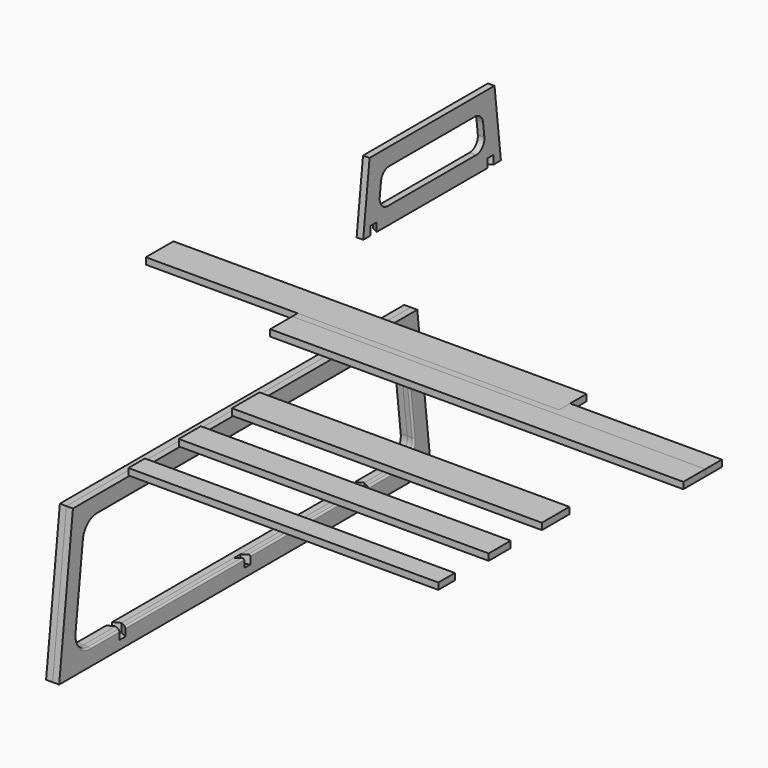
from build123d import *

# Parameters (mm, degrees)
F0_W          = 1200
F0_H          = 60
F1_DEPTH      = 19
F2_W          = 1200
F2_H          = 80
F3_DEPTH      = 19
F4_W          = 1200
F4_H          = 100
F5_DEPTH      = 19
F7_DEPTH      = 19
F8_DEPTH      = 19
F10_DEPTH     = 25
F12_DEPTH     = 25
F14_DEPTH     = 25
F16_DEPTH     = 25
F18_R         = 6.35
F19_DEPTH     = 10
F20_R         = 3.1
F21_DEPTH     = 571.5798048431
F22_R         = 6.35
F22_R_2       = 3.1
F23_DEPTH     = 10
F24_R         = 6.35
F25_DEPTH     = 10
F27_DEPTH     = 25
F28_DEPTH     = 25
F30_DEPTH     = 19
F32_DEPTH     = 25
F33_W         = 900
F33_H         = 60
F34_DEPTH     = 19
F33_H_2       = 80
F35_DEPTH     = 19
F33_H_3       = 100
F36_DEPTH     = 19
F37_T1_DEPTH  = 456.85740495
F37_T3_DEPTH  = 429.8821422275
F37_T5_DEPTH  = 128.89740651
F37_T7_DEPTH  = 118.9306462831
F37_T9_DEPTH  = 231.5496739088
F37_T11_DEPTH = 1071.9082714241
F37_T13_DEPTH = 231.5496739088
F37_T16_ANGLE = 96.6325146151
F37_T18_ANGLE = 83.3674853849
F37_T20_ANGLE = 83.3674853849
F37_T22_ANGLE = 96.6325146151


# Not quite as in the source:
# - a fillet or chamfer that OpenCascade refuses, or shapes differently, is made with other operations: its cross-section is extruded or revolved along the edge and cut away or added
# - a feature names something its author has since deleted; it is built from what else it names


with BuildPart() as f1:
    # F0 (on Top) → F1 (new body)
    with BuildSketch(Plane.XY):
        with Locations((600, 30)):
            Rectangle(F0_W, F0_H)
    extrude(amount=F1_DEPTH)

    # F24 (on face) → F25 (cut)
    with BuildSketch(Plane(origin=(0, 0, -182.5788048431), x_dir=(1, 0, 0), z_dir=(0, 0, -1))):
        with Locations((9.5, 194.6265311424)):
            Circle(F24_R)
    extrude(amount=-F25_DEPTH, mode=Mode.SUBTRACT)


with BuildPart() as f3:
    # F2 (on Top) → F3 (new body)
    with BuildSketch(Plane.XY):
        with Locations((600, -40)):
            Rectangle(F2_W, F2_H)
    extrude(amount=F3_DEPTH)


with BuildPart() as f5:
    # F4 (on Top) → F5 (new body)
    with BuildSketch(Plane.XY):
        with Locations((159.0859787539, 69.8453307072)):
            Rectangle(F4_W, F4_H)
    extrude(amount=F5_DEPTH)


with BuildPart() as f7:
    # F6 (on Right) → F7 (new body)
    with BuildSketch(Plane.YZ):
        Polygon((430.3734688576, -132.5788048431), (-819.6265311424, -132.5788048431), (-869.6265311424, -562.5788048431), (480.3734688576, -562.5788048431), align=None)
        with BuildLine():
            ThreePointArc((-780.2460358695, -226.8037619344), (-763.8315905601, -195.2374594909), (-730.5806668544, -182.5788048431))
            Line((-730.5806668544, -182.5788048431), (341.3276045696, -182.5788048431))
            ThreePointArc((341.3276045696, -182.5788048431), (374.5785282753, -195.2374594909), (390.9929735847, -226.8037619344))
            Line((390.9929735847, -226.8037619344), (417.7371596312, -456.8037619344))
            ThreePointArc((417.7371596312, -456.8037619344), (405.4131359684, -495.8297285488), (368.0717906162, -512.5788048431))
            Line((368.0717906162, -512.5788048431), (-757.3248529009, -512.5788048431))
            ThreePointArc((-757.3248529009, -512.5788048431), (-794.6661982532, -495.8297285488), (-806.990221916, -456.8037619344))
            Line((-806.990221916, -456.8037619344), (-780.2460358695, -226.8037619344))
        make_face(mode=Mode.SUBTRACT)
    extrude(amount=F7_DEPTH)

    # F9 (on face) → F10 (cut)
    with BuildSketch(Plane.XY.offset(-132.5788048431)):
        Polygon((19, -176.7615311424), (0, -189.5771929624), (0, -212.495333984), (19, -199.679672164), align=None)
    extrude(amount=-F10_DEPTH, mode=Mode.SUBTRACT)

    # F11 (on face) → F12 (cut)
    with BuildSketch(Plane.XY.offset(-512.5788048431)):
        Polygon((45.0043368484, -157.1230627047), (-59.9762402534, -227.9333560629), (-53.8986982225, -246.7521432232), (55.6290020144, -172.8747765833), align=None)
    extrude(amount=-F12_DEPTH, mode=Mode.SUBTRACT)

    # F18 (on face) → F19 (cut)
    with BuildSketch(Plane(origin=(0, 0, -562.5788048431), x_dir=(1, 0, 0), z_dir=(0, 0, -1))):
        with Locations((9.5, 194.6265311424)):
            Circle(F18_R)
    extrude(amount=-F19_DEPTH, mode=Mode.SUBTRACT)

    # F20 (on face) → F21 (cut, through all)
    with BuildSketch(Plane(origin=(0, 0, -552.5788048431), x_dir=(1, 0, 0), z_dir=(0, 0, -1))):
        with Locations((9.5, 194.6265311424)):
            Circle(F20_R)
    extrude(amount=-F21_DEPTH, mode=Mode.SUBTRACT)

    # F22 (on face) → F23 (cut)
    with BuildSketch(Plane(origin=(0, 0, -182.5788048431), x_dir=(1, 0, 0), z_dir=(0, 0, -1))):
        with Locations((9.5, 194.6265311424)):
            Circle(F22_R)
        with Locations((9.5, 194.6265311424)):
            Circle(F22_R_2, mode=Mode.SUBTRACT)
    extrude(amount=-F23_DEPTH, mode=Mode.SUBTRACT)


with BuildPart() as f8:
    # F6 (on Right) → F8 (new body)
    with BuildSketch(Plane.YZ):
        Polygon((430.3734688576, -132.5788048431), (-819.6265311424, -132.5788048431), (-869.6265311424, -562.5788048431), (480.3734688576, -562.5788048431), align=None)
        with BuildLine():
            ThreePointArc((-780.2460358695, -226.8037619344), (-763.8315905601, -195.2374594909), (-730.5806668544, -182.5788048431))
            Line((-730.5806668544, -182.5788048431), (341.3276045696, -182.5788048431))
            ThreePointArc((341.3276045696, -182.5788048431), (374.5785282753, -195.2374594909), (390.9929735847, -226.8037619344))
            Line((390.9929735847, -226.8037619344), (417.7371596312, -456.8037619344))
            ThreePointArc((417.7371596312, -456.8037619344), (405.4131359684, -495.8297285488), (368.0717906162, -512.5788048431))
            Line((368.0717906162, -512.5788048431), (-757.3248529009, -512.5788048431))
            ThreePointArc((-757.3248529009, -512.5788048431), (-794.6661982532, -495.8297285488), (-806.990221916, -456.8037619344))
            Line((-806.990221916, -456.8037619344), (-780.2460358695, -226.8037619344))
        make_face(mode=Mode.SUBTRACT)
    extrude(amount=-F8_DEPTH)

    # F13 (on face) → F14 (cut)
    with BuildSketch(Plane(origin=(0, 0, -562.5788048431), x_dir=(1, 0, 0), z_dir=(0, 0, -1))):
        Polygon((0, 212.4915311424), (-19, 199.6758693224), (-19, 176.7577283008), (0, 189.5733901208), align=None)
    extrude(amount=-F14_DEPTH, mode=Mode.SUBTRACT)

    # F15 (on face) → F16 (cut)
    with BuildSketch(Plane(origin=(0, 0, -182.5788048431), x_dir=(1, 0, 0), z_dir=(0, 0, -1))):
        Polygon((0, 212.4915311424), (-19, 199.6758693224), (-19, 176.7577283008), (0, 189.5733901208), align=None)
    extrude(amount=-F16_DEPTH, mode=Mode.SUBTRACT)


with BuildPart() as f27_tool:
    # F26 (on face) → F27 (new body)
    with BuildSketch(Plane.XY.offset(-512.5788048431)):
        Polygon((0, -619.4719911424), (0, -640.9274424049), (19, -650.8942066179), (19, -629.4387553554), align=None)
        Polygon((-87.6130647374, -686.8863244162), (0, -640.9274424049), (0, -619.4719911424), (-87.6130647374, -665.4308731537), align=None)
        Polygon((0, 261.6411483192), (0, 240.1856970567), (19, 230.2189328437), (19, 251.6743841062), align=None)
    extrude(amount=-F27_DEPTH)


with BuildPart() as f7_1:
    add(f7.part)

    # F27: cut by f27_tool
    add(f27_tool.part, mode=Mode.SUBTRACT)

    # F37: fillet of radius 5 on 11 edges, made by hand

    # F37_s2 → F37_t1 (cut)
    with BuildSketch(Plane.XZ.offset(185.0813504054)):
        with BuildLine():
            ThreePointArc((19, -517.5788048431), (17.5355339059, -514.0432709372), (14, -512.5788048431))
            Line((14, -512.5788048431), (19, -512.5788048431))
            Line((19, -512.5788048431), (19, -517.5788048431))
        make_face()
    extrude(amount=F37_T1_DEPTH, mode=Mode.SUBTRACT)

    # F37_s4 → F37_t3 (cut)
    with BuildSketch(Plane.XZ.offset(-242.7189328437)):
        with BuildLine():
            ThreePointArc((19, -517.5788048431), (17.5355339059, -514.0432709372), (14, -512.5788048431))
            Line((14, -512.5788048431), (19, -512.5788048431))
            Line((19, -512.5788048431), (19, -517.5788048431))
        make_face()
    extrude(amount=F37_T3_DEPTH, mode=Mode.SUBTRACT)

    # F37_s6 → F37_t5 (cut)
    with BuildSketch(Plane.XZ.offset(-368.0717906162)):
        with BuildLine():
            ThreePointArc((19, -517.5788048431), (17.5355339059, -514.0432709372), (14, -512.5788048431))
            Line((14, -512.5788048431), (19, -512.5788048431))
            Line((19, -512.5788048431), (19, -517.5788048431))
        make_face()
    extrude(amount=F37_T5_DEPTH, mode=Mode.SUBTRACT)

    # F37_s8 → F37_t7 (cut)
    with BuildSketch(Plane.XZ.offset(638.3942066179)):
        with BuildLine():
            ThreePointArc((19, -517.5788048431), (17.5355339059, -514.0432709372), (14, -512.5788048431))
            Line((14, -512.5788048431), (19, -512.5788048431))
            Line((19, -512.5788048431), (19, -517.5788048431))
        make_face()
    extrude(amount=F37_T7_DEPTH, mode=Mode.SUBTRACT)

    # F37_s10 → F37_t9 (cut)
    with BuildSketch(Plane(origin=(0, 31.2367306059, -268.635883211), x_dir=(1, 0, 0), z_dir=(0, 0.1155008582, -0.9933073803))):
        with BuildLine():
            ThreePointArc((19, -367.180177167), (17.5355339059, -363.644643261), (14, -362.180177167))
            Line((14, -362.180177167), (19, -362.180177167))
            Line((19, -362.180177167), (19, -367.180177167))
        make_face()
    extrude(amount=F37_T9_DEPTH, mode=Mode.SUBTRACT)

    # F37_s12 → F37_t11 (cut)
    with BuildSketch(Plane.XZ.offset(-341.3276045696)):
        with BuildLine():
            ThreePointArc((19, -177.5788048431), (17.5355339059, -181.1143387491), (14, -182.5788048431))
            Line((14, -182.5788048431), (19, -182.5788048431))
            Line((19, -182.5788048431), (19, -177.5788048431))
        make_face()
    extrude(amount=F37_T11_DEPTH, mode=Mode.SUBTRACT)

    # F37_s14 → F37_t13 (cut)
    with BuildSketch(Plane(origin=(0, -63.1737269817, -543.294052043), x_dir=(1, 0, 0), z_dir=(0, 0.1155008582, 0.9933073803))):
        with BuildLine():
            ThreePointArc((19, -753.8281167393), (17.5355339059, -750.2925828334), (14, -748.8281167393))
            Line((14, -748.8281167393), (19, -748.8281167393))
            Line((19, -748.8281167393), (19, -753.8281167393))
        make_face()
    extrude(amount=F37_T13_DEPTH, mode=Mode.SUBTRACT)

    # F37_s15 → F37_t16 (revolve, cut)
    with BuildSketch(Plane(origin=(0, 57.9809166524, -498.635883211), x_dir=(1, 0, 0), z_dir=(0, -0.1155008582, 0.9933073803))):
        with BuildLine():
            ThreePointArc((19, 367.180177167), (17.5355339059, 363.644643261), (14, 362.180177167))
            Line((14, 362.180177167), (19, 362.180177167))
            Line((19, 362.180177167), (19, 367.180177167))
        make_face()
    revolve(axis=Axis((19, 368.0717906162, -462.5788048431), (-1, 0, 0)), revolution_arc=F37_T16_ANGLE, mode=Mode.SUBTRACT)

    # F37_s17 → F37_t18 (revolve, cut)
    with BuildSketch(Plane.XZ.offset(-341.3276045696)):
        with BuildLine():
            ThreePointArc((19, -177.5788048431), (17.5355339059, -181.1143387491), (14, -182.5788048431))
            Line((14, -182.5788048431), (19, -182.5788048431))
            Line((19, -182.5788048431), (19, -177.5788048431))
        make_face()
    revolve(axis=Axis((19, 341.3276045696, -232.5788048431), (-1, 0, 0)), revolution_arc=F37_T18_ANGLE, mode=Mode.SUBTRACT)

    # F37_s19 → F37_t20 (revolve, cut)
    with BuildSketch(Plane(origin=(0, -36.4295409352, -313.294052043), x_dir=(1, 0, 0), z_dir=(0, -0.1155008582, -0.9933073803))):
        with BuildLine():
            ThreePointArc((19, 753.8281167393), (17.5355339059, 750.2925828334), (14, 748.8281167393))
            Line((14, 748.8281167393), (19, 748.8281167393))
            Line((19, 748.8281167393), (19, 753.8281167393))
        make_face()
    revolve(axis=Axis((19, -730.5806668544, -232.5788048431), (-1, 0, 0)), revolution_arc=F37_T20_ANGLE, mode=Mode.SUBTRACT)

    # F37_s21 → F37_t22 (revolve, cut)
    with BuildSketch(Plane.XZ.offset(757.3248529009)):
        with BuildLine():
            ThreePointArc((19, -517.5788048431), (17.5355339059, -514.0432709372), (14, -512.5788048431))
            Line((14, -512.5788048431), (19, -512.5788048431))
            Line((19, -512.5788048431), (19, -517.5788048431))
        make_face()
    revolve(axis=Axis((19, -757.3248529009, -462.5788048431), (-1, 0, 0)), revolution_arc=F37_T22_ANGLE, mode=Mode.SUBTRACT)


with BuildPart() as f8_1:
    add(f8.part)

    # F27: cut by f27_tool
    add(f27_tool.part, mode=Mode.SUBTRACT)

    # F26 (on face) → F28 (cut)
    with BuildSketch(Plane.XY.offset(-512.5788048431)):
        Polygon((0, -619.4719911424), (0, -640.9274424049), (87.6130647374, -686.8863244162), (87.6130647374, -665.4308731537), align=None)
        Polygon((-87.6130647374, -686.8863244162), (0, -640.9274424049), (0, -619.4719911424), (-87.6130647374, -665.4308731537), align=None)
        Polygon((0, 261.6411483192), (0, 240.1856970567), (19, 230.2189328437), (19, 251.6743841062), align=None)
        Polygon((-19, 230.2189328437), (0, 240.1856970567), (0, 261.6411483192), (-19, 251.6743841062), align=None)
    extrude(amount=-F28_DEPTH, mode=Mode.SUBTRACT)


with BuildPart() as f30:
    # F29 (on Right) → F30 (new body)
    with BuildSketch(Plane.YZ):
        Polygon((257.1804102281, 326.0098321468), (233.9334925731, 126.0098321468), (733.9334925731, 126.0098321468), (710.6865749182, 326.0098321468), align=None)
        with BuildLine():
            Line((328.4202492434, 276.0098321468), (639.4467359028, 276.0098321468))
            ThreePointArc((639.4467359028, 276.0098321468), (659.3977817761, 268.4142015546), (669.2461093573, 249.4735500511))
            Line((669.2461093573, 249.4735500511), (673.8954928883, 209.4735500511))
            ThreePointArc((673.8954928883, 209.4735500511), (666.5004888417, 186.0587862735), (644.0961194338, 176.0098321468))
            Line((644.0961194338, 176.0098321468), (323.7708657124, 176.0098321468))
            ThreePointArc((323.7708657124, 176.0098321468), (301.3664963045, 186.0587862735), (293.9714922579, 209.4735500511))
            Line((293.9714922579, 209.4735500511), (298.6208757889, 249.4735500511))
            ThreePointArc((298.6208757889, 249.4735500511), (308.4692033701, 268.4142015546), (328.4202492434, 276.0098321468))
        make_face(mode=Mode.SUBTRACT)
    extrude(amount=F30_DEPTH)

    # F31 (on face) → F32 (cut)
    with BuildSketch(Plane(origin=(0, 0, 126.0098321468), x_dir=(1, 0, 0), z_dir=(0, 0, -1))):
        Polygon((19, -282.7939438356), (19, -261.3384925731), (0, -271.3052567861), (0, -292.7607080486), align=None)
        Polygon((19, -706.5284925731), (19, -685.0730413106), (0, -675.1062770976), (0, -696.5617283601), align=None)
    extrude(amount=-F32_DEPTH, mode=Mode.SUBTRACT)


with BuildPart() as f34:
    # F33 (on Top) → F34 (new body)
    with BuildSketch(Plane.XY):
        with Locations((624.9209493399, -783.1725859803)):
            Rectangle(F33_W, F33_H)
    extrude(amount=F34_DEPTH)


with BuildPart() as f35:
    # F33 (on Top) → F35 (new body)
    with BuildSketch(Plane.XY):
        with Locations((624.9209493399, -590.4139791311)):
            Rectangle(F33_W, F33_H_2)
    extrude(amount=F35_DEPTH)


with BuildPart() as f36:
    # F33 (on Top) → F36 (new body)
    with BuildSketch(Plane.XY):
        with Locations((624.9209493399, -387.3105144983)):
            Rectangle(F33_W, F33_H_3)
    extrude(amount=F36_DEPTH)


solid = Compound([f1.part, f3.part, f5.part, f7_1.part, f8_1.part, f30.part, f34.part, f35.part, f36.part])
